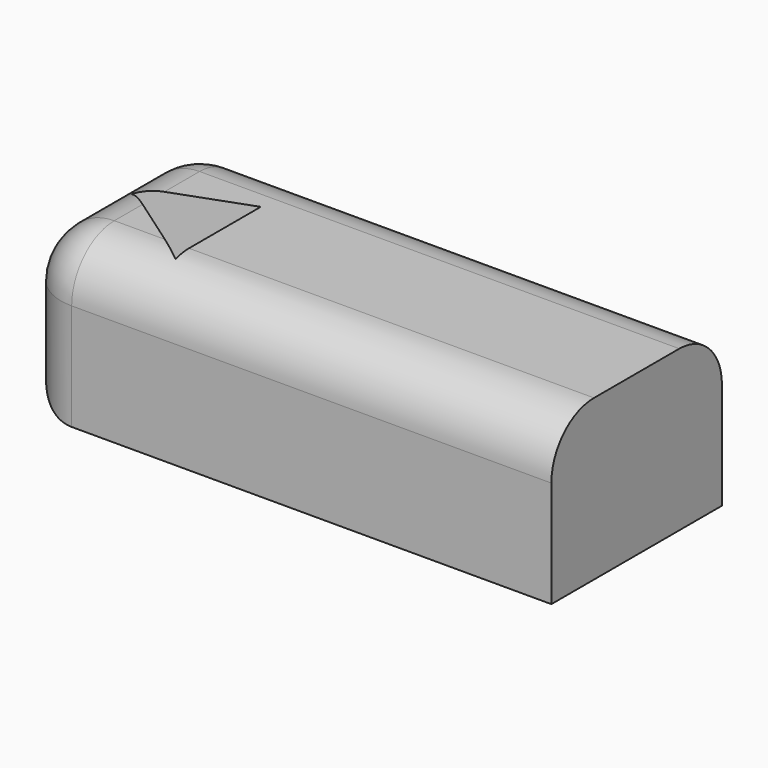
from build123d import *

# Parameters (mm, degrees)
F0_W         = 127
F0_H         = 50.8
F1_DEPTH     = 38.1
F2_T1_DEPTH  = 57.15
F2_T3_DEPTH  = 114.3
F2_T5_DEPTH  = 25.4
F2_T7_DEPTH  = 146.05
F2_S11_W     = 12.7
F2_S11_H     = 12.7
F2_T12_DEPTH = 12.7
F2_S17_W     = 12.7
F2_S17_H     = 12.7
F2_T18_DEPTH = 12.7


# Not quite as in the source:
# - a fillet or chamfer that OpenCascade refuses, or shapes differently, is made with other operations: its cross-section is extruded or revolved along the edge and cut away or added


with BuildPart() as f1:
    # F0 (on Top) → F1 (new body)
    with BuildSketch(Plane.XY):
        with Locations((4.3936092407, 0)):
            Rectangle(F0_W, F0_H)
        Polygon((-28.6239193533, -16.7126883595), (-52.4921119213, 0), (-28.6239193533, 8.6873116405), align=None, mode=Mode.SUBTRACT)
    extrude(amount=F1_DEPTH)

    # F2: fillet of radius 12.7 on 6 edges, made by hand

    # F2_s2 → F2_t1 (cut)
    with BuildSketch(Plane.XY.offset(-31.75)):
        with BuildLine():
            ThreePointArc((-46.4063907593, 25.4), (-55.3866468804, 21.6802561211), (-59.1063907593, 12.7))
            Line((-59.1063907593, 12.7), (-59.1063907593, 25.4))
            Line((-59.1063907593, 25.4), (-46.4063907593, 25.4))
        make_face()
        with BuildLine():
            ThreePointArc((-59.1063907593, -12.7), (-55.3866468804, -21.6802561211), (-46.4063907593, -25.4))
            Line((-46.4063907593, -25.4), (-59.1063907593, -25.4))
            Line((-59.1063907593, -25.4), (-59.1063907593, -12.7))
        make_face()
    extrude(amount=F2_T1_DEPTH, mode=Mode.SUBTRACT)

    # F2_s4 → F2_t3 (cut)
    with BuildSketch(Plane.XZ.offset(-57.15)):
        with BuildLine():
            ThreePointArc((-59.1063907593, 12.7), (-55.3866468804, 3.7197438789), (-46.4063907593, 0))
            Line((-46.4063907593, 0), (-59.1063907593, 0))
            Line((-59.1063907593, 0), (-59.1063907593, 12.7))
        make_face()
    extrude(amount=F2_T3_DEPTH, mode=Mode.SUBTRACT)

    # F2_s6 → F2_t5 (cut)
    with BuildSketch(Plane.XZ.offset(-12.7)):
        with BuildLine():
            ThreePointArc((-59.1063907593, 25.4), (-55.3866468804, 34.3802561211), (-46.4063907593, 38.1))
            Line((-46.4063907593, 38.1), (-59.1063907593, 38.1))
            Line((-59.1063907593, 38.1), (-59.1063907593, 25.4))
        make_face()
    extrude(amount=F2_T5_DEPTH, mode=Mode.SUBTRACT)

    # F2_s8 → F2_t7 (cut)
    with BuildSketch(Plane.YZ.offset(-46.4063907593)):
        with BuildLine():
            ThreePointArc((-25.4, 25.4), (-21.6802561211, 34.3802561211), (-12.7, 38.1))
            Line((-12.7, 38.1), (-25.4, 38.1))
            Line((-25.4, 38.1), (-25.4, 25.4))
        make_face()
        with BuildLine():
            ThreePointArc((25.4, 25.4), (21.6802561211, 34.3802561211), (12.7, 38.1))
            Line((12.7, 38.1), (25.4, 38.1))
            Line((25.4, 38.1), (25.4, 25.4))
        make_face()
    extrude(amount=F2_T7_DEPTH, mode=Mode.SUBTRACT)


with BuildPart() as f2_tool10:
    # F2_s11 → F2_t12 (new body)
    with BuildSketch(Plane.XZ.offset(-12.7)):
        with Locations((-52.7563907593, 31.75)):
            Rectangle(F2_S11_W, F2_S11_H)
    extrude(amount=-F2_T12_DEPTH)

    # F2_s13 → F2_t14 (revolve, cut)
    with BuildSketch(Plane(origin=(-46.4063907593, 12.7, 25.4), x_dir=(0.7071067812, 0, -0.7071067812), z_dir=(0.7071067812, 0, 0.7071067812))):
        with BuildLine():
            ThreePointArc((0, -12.7), (12.7, 0), (0, 12.7))
            Line((0, 12.7), (0, -12.7))
        make_face()
    revolve(axis=Axis((-46.4063907593, 12.7, 25.4), (0, 1, 0)), mode=Mode.SUBTRACT)


with BuildPart() as f1_1:
    add(f1.part)

    # F2_t9: cut F2_tool10
    add(f2_tool10.part, mode=Mode.SUBTRACT)


with BuildPart() as f2_tool16:
    # F2_s17 → F2_t18 (new body)
    with BuildSketch(Plane.XY.offset(25.4)):
        with Locations((-52.7563907593, -19.05)):
            Rectangle(F2_S17_W, F2_S17_H)
    extrude(amount=F2_T18_DEPTH)

    # F2_s19 → F2_t20 (revolve, cut)
    with BuildSketch(Plane(origin=(-46.4063907593, -12.7, 25.4), x_dir=(0.7071067812, 0.7071067812, 0), z_dir=(0.7071067812, -0.7071067812, 0))):
        with BuildLine():
            ThreePointArc((0, -12.7), (12.7, 0), (0, 12.7))
            Line((0, 12.7), (0, -12.7))
        make_face()
    revolve(axis=Axis((-46.4063907593, -12.7, 25.4), (0, 0, 1)), mode=Mode.SUBTRACT)


with BuildPart() as f1_2:
    add(f1_1.part)

    # F2_t15: cut F2_tool16
    add(f2_tool16.part, mode=Mode.SUBTRACT)


solid = f1_2.part
